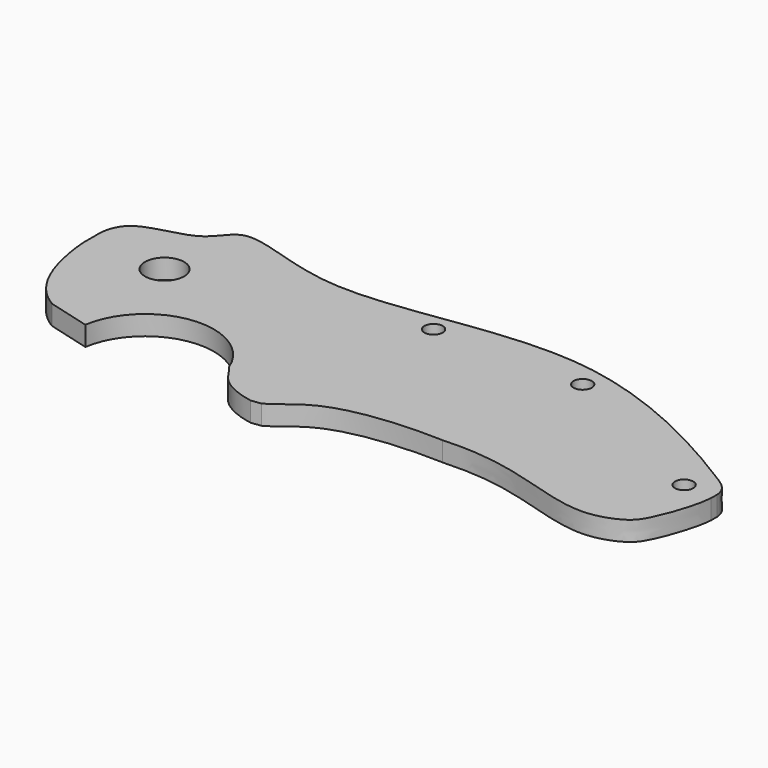
from build123d import *

# Parameters (mm, degrees)
F0_W      = 127
F0_H      = 76.2
F1_DEPTH  = 3.81
F3_DEPTH  = 3.811
F5_DEPTH  = 3.8110001
F7_DEPTH  = 3.8110001
F9_DEPTH  = 3.8110001
F11_DEPTH = 3.8110001
F12_R     = 3.81
F12_R_2   = 1.778
F13_DEPTH = 3.8110001


# Not quite as in the source:
# - a feature names something its author has since deleted; it is built from what else it names


with BuildPart() as f1:
    # F0 (on Top) → F1 (new body)
    with BuildSketch(Plane.XY):
        Rectangle(F0_W, F0_H)
    extrude(amount=F1_DEPTH)

    # F2 (on face) → F3 (cut, through all)
    with BuildSketch(Plane.XY.offset(3.81)):
        with BuildLine():
            add(Edge.make_bspline(
                [(63.5, 10.6295113671), (63.2612207711, 7.3334525683), (60.4792156138, -0.6175861792), (57.8984243973, -3.4201330935), (51.0670932701, -5.9462304059), (40.4260203479, -3.1372131349), (25.9703202997, 1.5196992045), (1.8583117509, -1.8157493622), (-5.3459736097, -9.8899644198), (-19.0690661476, -6.4890316998), (-20.4937441159, 2.1095905456), (-40.7770743847, 1.977731645), (-43.545073038, -6.2710383318), (-60.2821322563, -1.8131008621), (-63.0791562706, 11.1616425579), (-63.5, 16.6433006525)],
                knots=[0.4059955099, 0.4059955099, 0.4059955099, 0.4059955099, 0.4476692289, 0.4757284115, 0.5102067466, 0.5545414454, 0.6089875876, 0.6747122657, 0.7184103973, 0.7643733792, 0.8011148978, 0.857072106, 0.8928624664, 0.9424351499, 1, 1, 1, 1], degree=3))
            Line((-63.5, 16.6433006525), (-63.5, -38.1))
            Line((-63.5, -38.1), (63.5, -38.1))
            Line((63.5, -38.1), (63.5, 10.6295113671))
        make_face()
        with BuildLine():
            Line((-63.5, 38.1), (-63.5, 20.9406016115))
            add(Edge.make_bspline(
                [(-63.5, 20.9406016115), (-63.2705171092, 22.8756120124), (-61.4344823587, 27.3135037603), (-49.7373849082, 27.8474409075), (-46.6167172081, 37.1774806899), (-23.625240799, 24.3038333511), (20.2561645612, 40.5363242915), (58.3281350692, 17.4440815598), (63.2868268374, 14.3726929767), (63.5, 12.0625765994)],
                knots=[0.0164641001, 0.0164641001, 0.0164641001, 0.0164641001, 0.0412846178, 0.0868073878, 0.1215977861, 0.1830290889, 0.2770460049, 0.364414327, 0.3994411549, 0.3994411549, 0.3994411549, 0.3994411549], degree=3))
            Line((63.5, 12.0625765994), (63.5, 38.1))
            Line((63.5, 38.1), (-63.5, 38.1))
        make_face()
    extrude(amount=-F3_DEPTH, mode=Mode.SUBTRACT)

    # F4 (on face) → F5 (cut, through all)
    with BuildSketch(Plane.XY.offset(3.81)):
        with BuildLine():
            ThreePointArc((-20.6505600777, -1.4318204309), (-34.5910698398, 7.044758626), (-46.3664438914, -4.24819364))
            Line((-46.3664438914, -4.24819364), (-45.886389514, -4.3784275947))
            add(Edge.make_bspline(
                [(-20.6505600777, -1.4318204309), (-21.1230409062, -0.8987729822), (-24.5539183179, 2.0831959595), (-40.7770743847, 1.977731645), (-42.6866550388, -3.7129111407), (-45.471096336, -4.3272746905), (-45.886389514, -4.3784275947)],
                knots=[0.7900934198, 0.7900934198, 0.7900934198, 0.7900934198, 0.8011148978, 0.857072106, 0.8928624664, 0.8986085939, 0.8986085939, 0.8986085939, 0.8986085939], degree=3))
        make_face()
        with BuildLine():
            Line((-46.3664438914, -4.24819364), (-54.6990786485, -1.9876331092))
            add(Edge.make_bspline(
                [(-46.3918791935, -4.4232407036), (-48.769167695, -4.556578226), (-51.9448590774, -3.7018502861), (-54.6990786485, -1.9876331092)],
                knots=[0.9008772209, 0.9008772209, 0.9008772209, 0.9008772209, 0.9320742237, 0.9320742237, 0.9320742237, 0.9320742237], degree=3))
            ThreePointArc((-46.3918791935, -4.4232407036), (-46.3794507135, -4.3356751536), (-46.3664438914, -4.24819364))
        make_face()
    extrude(amount=-F5_DEPTH, mode=Mode.SUBTRACT)

    # F6 (on face) → F7 (cut, through all)
    with BuildSketch(Plane.XY.offset(3.81)):
        with BuildLine():
            add(Edge.make_bspline(
                [(-10.2358234775, -8.15383402), (-7.802055898, -7.3862587687), (-2.9799970638, -1.0143147696), (11.5796876732, 0.3192890418), (19.767615732, 0)],
                knots=[0.1496918409, 0.1496918409, 0.1496918409, 0.1496918409, 0.2257791994, 0.3455194422, 0.3455194422, 0.3455194422, 0.3455194422], degree=3))
            add(Edge.make_bspline(
                [(19.767615732, 0), (13.532714249, -0.3050525246), (1.1246225544, -2.6380327757), (-3.891051062, -8.2593575026), (-8.9495830463, -8.3000062317), (-10.2358234775, -8.15383402)],
                knots=[0.6248121796, 0.6248121796, 0.6248121796, 0.6248121796, 0.6747122657, 0.7184103973, 0.7329928494, 0.7329928494, 0.7329928494, 0.7329928494], degree=3))
        make_face()
    extrude(amount=-F7_DEPTH, mode=Mode.SUBTRACT)

    # F8 (on face) → F9 (cut, through all)
    with BuildSketch(Plane.XY.offset(3.81)):
        with BuildLine():
            Line((-9.3076174304, -7.7717970049), (-11.1768481928, -8.0197561819))
            add(Edge.make_bspline(
                [(-10.2358234775, -8.15383402), (-10.5488919391, -8.1182559832), (-10.8631772032, -8.0734157773), (-11.1768481928, -8.0197561819)],
                knots=[0.7329928494, 0.7329928494, 0.7329928494, 0.7329928494, 0.7365421903, 0.7365421903, 0.7365421903, 0.7365421903], degree=3))
            add(Edge.make_bspline(
                [(-10.2358234775, -8.15383402), (-9.9183933726, -8.0537211355), (-9.6104928812, -7.924549578), (-9.3076174304, -7.7717970049)],
                knots=[0.1496918409, 0.1496918409, 0.1496918409, 0.1496918409, 0.1596157213, 0.1596157213, 0.1596157213, 0.1596157213], degree=3))
        make_face()
    extrude(amount=-F9_DEPTH, mode=Mode.SUBTRACT)

    # F10 (on face) → F11 (cut, through all)
    with BuildSketch(Plane.XY.offset(3.81)):
        with BuildLine():
            Line((-46.4481910946, -4.2260164407), (-47.8414706886, -5.2504870109))
            Line((-47.8414706886, -5.2504870109), (-44.371560216, -5.1484312862))
            Line((-44.371560216, -5.1484312862), (-44.371560216, -2.6990815531))
            Line((-44.371560216, -2.6990815531), (-46.351980308, -4.1552731959))
            ThreePointArc((-46.351980308, -4.1552731959), (-46.3592937063, -4.2017207154), (-46.3664438914, -4.24819364))
            Line((-46.3664438914, -4.24819364), (-46.4481910946, -4.2260164407))
        make_face()
    extrude(amount=-F11_DEPTH, mode=Mode.SUBTRACT)

    # F12 (on face) → F13 (cut, through all)
    with BuildSketch(Plane.XY.offset(3.81)):
        with Locations((-48.4029985964, 17.5594463944)):
            Circle(F12_R)
        with Locations((-4.1226525791, 27.6370421052)):
            Circle(F12_R_2)
        with Locations((24.888606742, 27.6370421052)):
            Circle(F12_R_2)
        with Locations((57.56444484, 11.451812461)):
            Circle(F12_R_2)
    extrude(amount=-F13_DEPTH, mode=Mode.SUBTRACT)


solid = f1.part
